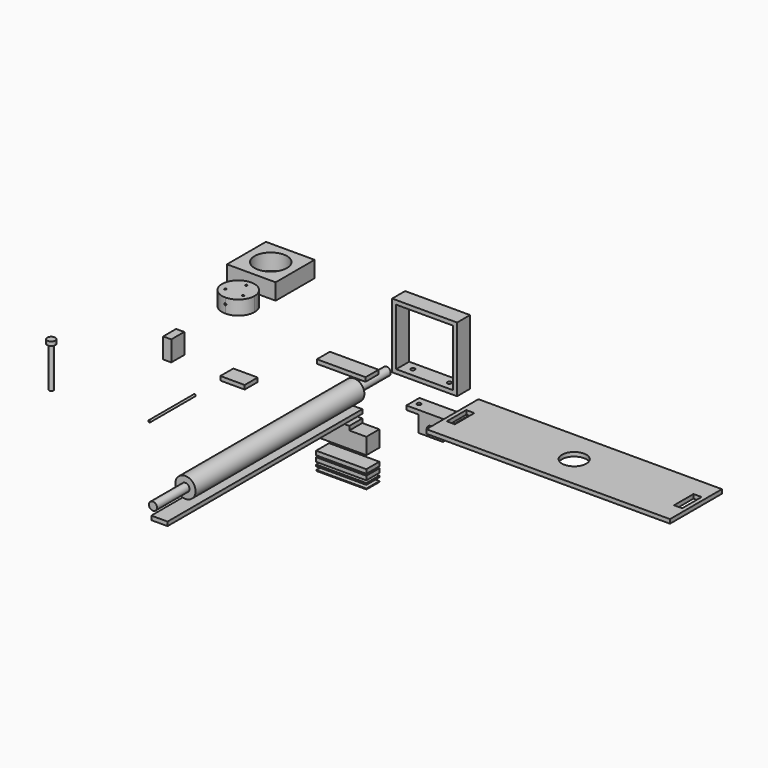
from build123d import *

# Parameters (mm, degrees)
F0_R      = 5
F1_DEPTH  = 20
F0_W      = 60
F0_H      = 5
F0_W_2    = 80
F0_H_2    = 80
F0_W_3    = 70
F0_H_3    = 70
F0_W_4    = 61.861140081
F0_H_4    = 1
F0_H_5    = 2
F0_R_2    = 12.5
F2_DEPTH  = 260
F3_R      = 5
F4_DEPTH  = 50
F5_DEPTH  = 300
F6_R      = 2.5
F7_DEPTH  = 25
F9_R      = 2.5
F8_R      = 2.5
F10_DEPTH = 25
F14_R     = 5
F15_DEPTH = 50
F16_W     = 300
F16_H     = 5
F17_DEPTH = 80
F20_DEPTH = 17.5
F19_W     = 60
F19_H     = 60
F19_R     = 20
F21_DEPTH = 20
F18_W     = 10
F18_H     = 30
F18_R     = 15
F22_DEPTH = 129.4251411048
F18_H_2   = 20
F23_DEPTH = 25
F18_W_2   = 30
F24_DEPTH = 5
F13_R     = 2.5
F25_DEPTH = 5
F26_R     = 5
F27_DEPTH = 5
F28_R     = 2.5
F29_DEPTH = 50
F32_DEPTH = 111.1712381574
F33_R     = 1.25
F34_DEPTH = 70
F35_R     = 1.25
F36_DEPTH = 107.1461310813


# Not quite as in the source:
# - a feature of the source that left no trace in its solid (it failed there, or was rolled back) is left out
# - a feature names something its author has since deleted; it is built from what else it names


with BuildPart() as f1:
    # F0 (on Front) → F1 (new body)
    with BuildSketch(Plane.XZ):
        Polygon((95.2936565876, -7.5), (110.2936565876, -7.5), (125.2936565876, -7.5), (125.2936565876, 12.5), (140.2936565876, 12.5), (140.2936565876, 17.5), (110.2936565876, 17.5), (80.2936565876, 17.5), (80.2936565876, 12.5), (95.2936565876, 12.5), align=None)
        with Locations((110.2936565876, 0)):
            Circle(F0_R, mode=Mode.SUBTRACT)
    extrude(amount=F1_DEPTH)

    # F9 (on face) + F8 (on face) → F10 (cut)
    with BuildSketch(Plane(origin=(0, 0, 12.5), x_dir=(1, 0, 0), z_dir=(0, 0, -1))):
        with Locations((87.7936565876, 10)):
            Circle(F9_R)
    with BuildSketch(Plane(origin=(0, 0, 12.5), x_dir=(1, 0, 0), z_dir=(0, 0, -1))):
        with Locations((132.7936565876, 10)):
            Circle(F8_R)
    extrude(amount=-F10_DEPTH, mode=Mode.SUBTRACT)


with BuildPart() as f1b:
    # F0 (on Front) → F1, piece 2 (new body)
    with BuildSketch(Plane.XZ):
        with Locations((0, 29.2427036911)):
            Rectangle(F0_W, F0_H)
    extrude(amount=F1_DEPTH)


with BuildPart() as f1c:
    # F0 (on Front) → F1, piece 3 (new body)
    with BuildSketch(Plane.XZ):
        Polygon((10, -27.5771580637), (0, -27.5771580637), (-10, -27.5771580637), (-10, -32.5771580637), (-10.9305700405, -32.5771580637), (-30.9305700405, -32.5771580637), (-30.9305700405, -52.5771580637), (0, -52.5771580637), (30.9305700405, -52.5771580637), (30.9305700405, -32.5771580637), (10.9305700405, -32.5771580637), (10, -32.5771580637), align=None)
    extrude(amount=F1_DEPTH)

    # F6 (on face) → F7 (cut)
    with BuildSketch(Plane.XY.offset(-32.5771580637)):
        with Locations((-20, -10)):
            Circle(F6_R)
    extrude(amount=-F7_DEPTH, mode=Mode.SUBTRACT)


with BuildPart() as f1d:
    # F0 (on Front) → F1, piece 4 (new body)
    with BuildSketch(Plane.XZ):
        with Locations((102.7326732874, 87.7068325877)):
            Rectangle(F0_W_2, F0_H_2)
        with Locations((102.7326732874, 87.7068325877)):
            Rectangle(F0_W_3, F0_H_3, mode=Mode.SUBTRACT)
    extrude(amount=F1_DEPTH)

    # F13 (on face) → F25 (cut, through all)
    with BuildSketch(Plane(origin=(0, 0, 47.7068325877), x_dir=(1, 0, 0), z_dir=(0, 0, -1))):
        with Locations((125.2326732874, 10)):
            Circle(F13_R)
        with Locations((80.2326732874, 10)):
            Circle(F13_R)
    extrude(amount=-F25_DEPTH, mode=Mode.SUBTRACT)


with BuildPart() as f1e:
    # F0 (on Front) → F1, piece 5 (new body)
    with BuildSketch(Plane.XZ):
        with Locations((0, -77.355325222)):
            Rectangle(F0_W_4, F0_H)
    extrude(amount=F1_DEPTH)


with BuildPart() as f1f:
    # F0 (on Front) → F1, piece 6 (new body)
    with BuildSketch(Plane.XZ):
        with Locations((0.1928325291, -89.1451310813)):
            Rectangle(F0_W_4, F0_H_4)
    extrude(amount=F1_DEPTH)


with BuildPart() as f1g:
    # F0 (on Front) → F1, piece 7 (new body)
    with BuildSketch(Plane.XZ):
        with Locations((0, -83.756296128)):
            Rectangle(F0_W_4, F0_H_5)
    extrude(amount=F1_DEPTH)


with BuildPart() as f1h:
    # F0 (on Front) → F1, piece 8 (new body)
    with BuildSketch(Plane.XZ):
        with Locations((0, -70.2389810979)):
            Rectangle(F0_W_4, F0_H)
    extrude(amount=F1_DEPTH)


with BuildPart() as f2:
    # F0 (on Front) → F2 (new body)
    with BuildSketch(Plane.XZ):
        Circle(F0_R_2)
    extrude(amount=F2_DEPTH)

    # F3 (on face) → F4 (join)
    with BuildSketch(Plane.XZ.offset(260)):
        Circle(F3_R)
    extrude(amount=F4_DEPTH)

    # F14 (on face) → F15 (join)
    with BuildSketch(Plane(origin=(0, 0, 0), x_dir=(-1, 0, 0), z_dir=(0, 1, 0))):
        Circle(F14_R)
    extrude(amount=F15_DEPTH)


with BuildPart() as f5:
    # F0 (on Front) → F5 (new body)
    with BuildSketch(Plane.XZ):
        Polygon((-10, -22.5167013705), (0, -22.5167013705), (10, -22.5167013705), (10, -17.5167013705), (0, -17.5167013705), (-10, -17.5167013705), align=None)
    extrude(amount=F5_DEPTH)


with BuildPart() as f17:
    # F16 (on Front) → F17 (new body)
    with BuildSketch(Plane.XZ):
        with Locations((303.0256081372, 37.2790100235)):
            Rectangle(F16_W, F16_H)
    extrude(amount=F17_DEPTH)

    # F18 (on face) → F22 (cut, through all)
    with BuildSketch(Plane.XY.offset(39.7790100235)):
        with Locations((163.0256081372, -40)):
            Rectangle(F18_W, F18_H)
        with Locations((443.0256081372, -40)):
            Rectangle(F18_W, F18_H)
        with Locations((303.0256081372, -40)):
            Circle(F18_R)
    extrude(amount=-F22_DEPTH, mode=Mode.SUBTRACT)


with BuildPart() as f20:
    # F19 (on Top) → F20 (new body)
    with BuildSketch(Plane.XY):
        with BuildLine():
            ThreePointArc((-196.265943614, 46.8016631402), (-182.1238079903, 52.6595275165), (-176.265943614, 66.8016631402))
            ThreePointArc((-176.265943614, 66.8016631402), (-210.4080792377, 80.9437987639), (-196.265943614, 46.8016631402))
        make_face()
    extrude(amount=F20_DEPTH)

    # F31 (on face) → F32 (cut, through all)
    with BuildSketch(Plane(origin=(0, 46.8016631402, 0), x_dir=(-1, 0, 0), z_dir=(0, 1, 0))):
        with BuildLine():
            Line((196.265943614, 8.75), (196.265943614, 11.25))
            ThreePointArc((196.265943614, 11.25), (195.015943614, 10), (196.265943614, 8.75))
        make_face()
        with BuildLine():
            ThreePointArc((196.265943614, 8.75), (197.1498270905, 9.1161165235), (197.515943614, 10))
            ThreePointArc((197.515943614, 10), (197.1498270905, 10.8838834765), (196.265943614, 11.25))
            Line((196.265943614, 11.25), (196.265943614, 8.75))
        make_face()
    extrude(amount=F32_DEPTH, mode=Mode.SUBTRACT)

    # F35 (on face) → F36 (cut, through all)
    with BuildSketch(Plane.XY.offset(17.5)):
        with Locations((-196.265943614, 79.3016631402)):
            Circle(F35_R)
        with Locations((-185.4406260667, 60.5516631402)):
            Circle(F35_R)
        with Locations((-207.0912611613, 60.5516631402)):
            Circle(F35_R)
    extrude(amount=-F36_DEPTH, mode=Mode.SUBTRACT)


with BuildPart() as f21:
    # F19 (on Top) → F21 (new body)
    with BuildSketch(Plane.XY):
        with Locations((-205.1943850517, 127.9719012976)):
            Rectangle(F19_W, F19_H)
        with Locations((-205.1943850517, 127.9719012976)):
            Circle(F19_R, mode=Mode.SUBTRACT)
    extrude(amount=F21_DEPTH)


with BuildPart() as f23:
    # F18 (on face) → F23 (new body)
    with BuildSketch(Plane.XY.offset(39.7790100235)):
        with Locations((-130.5344802141, -114.8494374752)):
            Rectangle(F18_W, F18_H_2)
    extrude(amount=F23_DEPTH)


with BuildPart() as f24:
    # F18 (on face) → F24 (new body)
    with BuildSketch(Plane.XY.offset(39.7790100235)):
        with Locations((-50.0688782334, -114.8494374752)):
            Rectangle(F18_W_2, F18_H_2)
    extrude(amount=F24_DEPTH)


with BuildPart() as f27:
    # F26 (on Top) → F27 (new body)
    with BuildSketch(Plane.XY):
        with Locations((-287.8777384163, -106.7102653366)):
            Circle(F26_R)
    extrude(amount=F27_DEPTH)

    # F28 (on face) → F29 (join)
    with BuildSketch(Plane.XY):
        with Locations((-287.7346277237, -106.8533882499)):
            Circle(F28_R)
    extrude(amount=-F29_DEPTH)


with BuildPart() as f34:
    # F33 (on Front) → F34 (new body)
    with BuildSketch(Plane.XZ):
        with Locations((-196.4730769396, -69.498129189)):
            Circle(F33_R)
    extrude(amount=F34_DEPTH)


solid = Compound([f1.part, f1b.part, f1c.part, f1d.part, f1e.part, f1f.part, f1g.part, f1h.part, f2.part, f5.part, f17.part, f20.part, f21.part, f23.part, f24.part, f27.part, f34.part])
